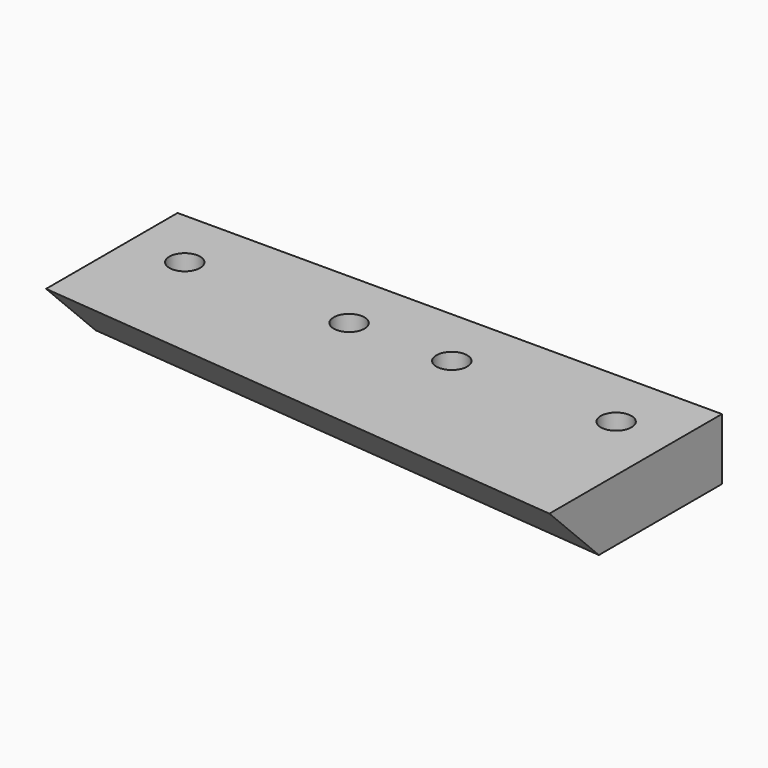
from build123d import *

# Parameters (mm, degrees)
F1_DEPTH = 6
F2_SIZE  = 5.99999
F3_R     = 1.5
F4_DEPTH = 6


# Not quite as in the source:
# - a fillet or chamfer is up to 0.001 mm smaller than in the source, because OpenCascade refuses the exact size


with BuildPart() as f1:
    # F0 (on Top) → F1 (new body)
    with BuildSketch(Plane.XY):
        Polygon((49.2662842423, 5.9127185345), (-3.7337157577, 5.9127185345), (-3.7337157577, -10.0872814655), (49.2662842423, -15.0872814655), align=None)
    extrude(amount=F1_DEPTH)

    # F2 (size 6 in the source; OpenCascade refuses exactly that, so slightly less here)
    f2_edges = [f1.edges().sort_by_distance(p)[0] for p in [
        (22.766284, -12.587281, 0),
    ]]
    chamfer(f2_edges, length=F2_SIZE)

    # F3 (on face) → F4 (cut, through all)
    with BuildSketch(Plane.XY.offset(6)):
        with Locations((1.7662842423, -0.0872814655)):
            Circle(F3_R)
        with Locations((17.7662842423, -0.0872814655)):
            Circle(F3_R)
        with Locations((27.7662842423, -0.0872814655)):
            Circle(F3_R)
        with Locations((43.7662842423, -0.0872814655)):
            Circle(F3_R)
    extrude(amount=-F4_DEPTH, mode=Mode.SUBTRACT)


solid = f1.part
